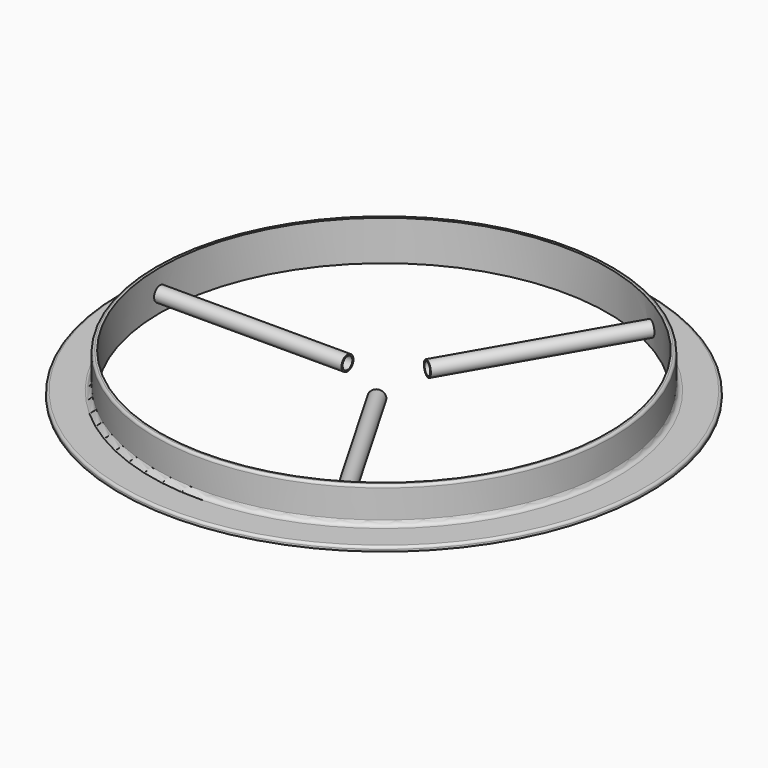
from build123d import *

# Parameters (mm, degrees)
F2_R            = 16.85
F2_R_2          = 13.65
F3_DEPTH        = 422
F3_COPIES_COUNT = 3


# Not quite as in the source:
# - a pattern or mirror of a feature is missing from the dataset's text; its kind, count and spacing are read off the source's solid


with BuildPart() as f1:
    # F0 (on Front) → F1 (revolve)
    with BuildSketch(Plane.XZ):
        with BuildLine():
            Line((-90, 4.5), (-90, 0))
            Line((-90, 0), (0, 0))
            Line((0, 0), (0, 90))
            Line((0, 90), (-4.5, 90))
            ThreePointArc((-4.5, 90), (-8.3890872965, 88.3890872965), (-10, 84.5))
            Line((-10, 84.5), (-10, 21))
            ThreePointArc((-10, 21), (-13.2218254069, 13.2218254069), (-21, 10))
            Line((-21, 10), (-84.5, 10))
            ThreePointArc((-84.5, 10), (-88.3890872965, 8.3890872965), (-90, 4.5))
        make_face()
    revolve(axis=Axis((504, 0, 45), (0, 0, 1)))

    # F2 (on Right) → F3 (join)
    with BuildSketch(Plane.YZ):
        with Locations((0, 38)):
            Circle(F2_R)
        with Locations((0, 38)):
            Circle(F2_R_2, mode=Mode.SUBTRACT)
    f3 = extrude(amount=F3_DEPTH)

    # F3_copies: F3 ×3 about axis
    f3_copies_axis = Axis((504.000031, 0, 0), (0, 0, 1))
    for i in range(1, F3_COPIES_COUNT):
        add(f3.rotate(f3_copies_axis, i * 360 / F3_COPIES_COUNT))


solid = f1.part
